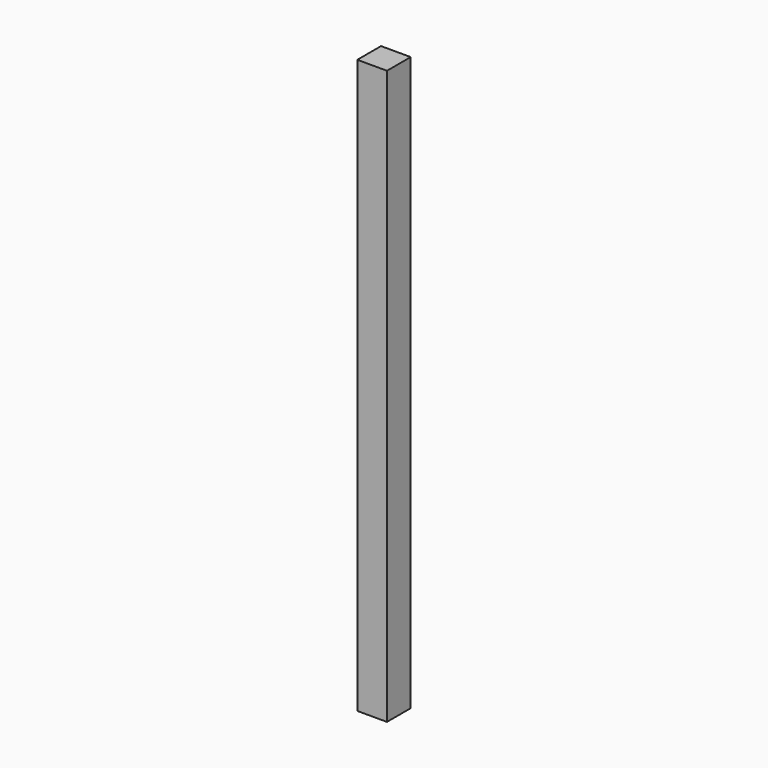
from build123d import *

# Parameters (mm, degrees)
F0_W     = 44
F0_H     = 44
F1_DEPTH = 850
F2_R     = 5
F3_DEPTH = 10
F4_R     = 5
F5_DEPTH = 10


# Not quite as in the source:
# - a feature names something its author has since deleted; it is built from what else it names


with BuildPart() as f1:
    # F0 (on Top) → F1 (new body)
    with BuildSketch(Plane.XY):
        with Locations((22, 22)):
            Rectangle(F0_W, F0_H)
    extrude(amount=F1_DEPTH)

    # F2 (on face) → F3 (cut)
    with BuildSketch(Plane(origin=(0, 44, 0), x_dir=(-1, 0, 0), z_dir=(0, 1, 0))):
        with Locations((-35, 115)):
            Circle(F2_R)
        with Locations((-35, 135)):
            Circle(F2_R)
        with Locations((-9, 435)):
            Circle(F2_R)
        with Locations((-35, 835)):
            Circle(F2_R)
        with Locations((-35, 815)):
            Circle(F2_R)
        with Locations((-9, 455)):
            Circle(F2_R)
    extrude(amount=-F3_DEPTH, mode=Mode.SUBTRACT)

    # F4 (on face) → F5 (cut)
    with BuildSketch(Plane(origin=(0, 0, 0), x_dir=(0, -1, 0), z_dir=(-1, 0, 0))):
        with Locations((-22, 135)):
            Circle(F4_R)
        with Locations((-22, 115)):
            Circle(F4_R)
        with Locations((-22, 838)):
            Circle(F4_R)
        with Locations((-22, 818)):
            Circle(F4_R)
    extrude(amount=-F5_DEPTH, mode=Mode.SUBTRACT)


solid = f1.part
